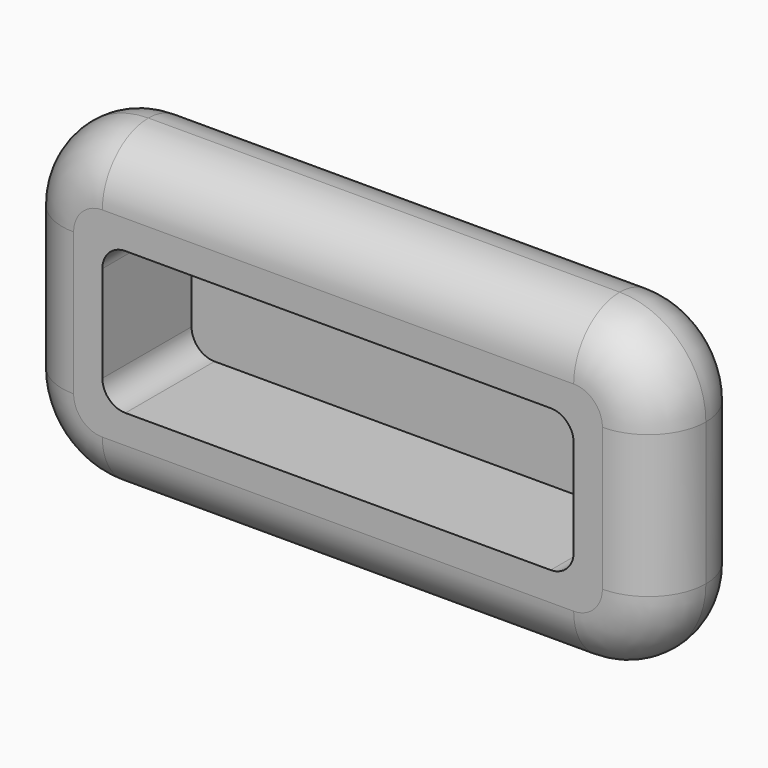
from build123d import *

# Parameters (mm, degrees)
F1_DEPTH = 20
F2_R     = 9.99999
F4_DEPTH = 19.4


# Not quite as in the source:
# - a fillet or chamfer is up to 0.001 mm smaller than in the source, because OpenCascade refuses the exact size


with BuildPart() as f1:
    # F0 (on Front) → F1 (new body)
    with BuildSketch(Plane.XZ):
        with BuildLine():
            ThreePointArc((55.998519063, 12.3981075734), (51.6051207808, 23.0047092912), (40.998519063, 27.3981075734))
            Line((40.998519063, 27.3981075734), (-40.998519063, 27.3981075734))
            ThreePointArc((-40.998519063, 27.3981075734), (-51.6051207808, 23.0047092912), (-55.998519063, 12.3981075734))
            Line((-55.998519063, 12.3981075734), (-55.998519063, -12.3981075734))
            ThreePointArc((-55.998519063, -12.3981075734), (-51.6051207808, -23.0047092912), (-40.998519063, -27.3981075734))
            Line((-40.998519063, -27.3981075734), (40.998519063, -27.3981075734))
            ThreePointArc((40.998519063, -27.3981075734), (51.6051207808, -23.0047092912), (55.998519063, -12.3981075734))
            Line((55.998519063, -12.3981075734), (55.998519063, 12.3981075734))
        make_face()
    extrude(amount=F1_DEPTH)

    # F2 (radius 10 in the source; OpenCascade refuses exactly that, so slightly less here)
    f2_edges = [f1.edges().sort_by_distance(p)[0] for p in [
        (55.998519, -20, 0),
        (51.605121, -20, 23.004709),
        (0, -20, 27.398108),
        (-51.605121, -20, 23.004709),
        (-55.998519, -20, 0),
        (-51.605121, -20, -23.004709),
        (0, -20, -27.398108),
        (51.605121, -20, -23.004709),
        (0, 0, 27.398108),
    ]]
    fillet(f2_edges, radius=F2_R)

    # F3 (on face) → F4 (cut)
    with BuildSketch(Plane.XZ.offset(20)):
        with BuildLine():
            ThreePointArc((-40.998519063, -8.3981075734), (-39.8269461877, -11.2265346981), (-36.998519063, -12.3981075734))
            Line((-36.998519063, -12.3981075734), (36.998519063, -12.3981075734))
            ThreePointArc((36.998519063, -12.3981075734), (39.8269461877, -11.2265346981), (40.998519063, -8.3981075734))
            Line((40.998519063, -8.3981075734), (40.998519063, 8.3981075734))
            ThreePointArc((40.998519063, 8.3981075734), (39.8269461877, 11.2265346981), (36.998519063, 12.3981075734))
            Line((36.998519063, 12.3981075734), (-36.998519063, 12.3981075734))
            ThreePointArc((-36.998519063, 12.3981075734), (-39.8269461877, 11.2265346981), (-40.998519063, 8.3981075734))
            Line((-40.998519063, 8.3981075734), (-40.998519063, -8.3981075734))
        make_face()
    extrude(amount=-F4_DEPTH, mode=Mode.SUBTRACT)


solid = f1.part
